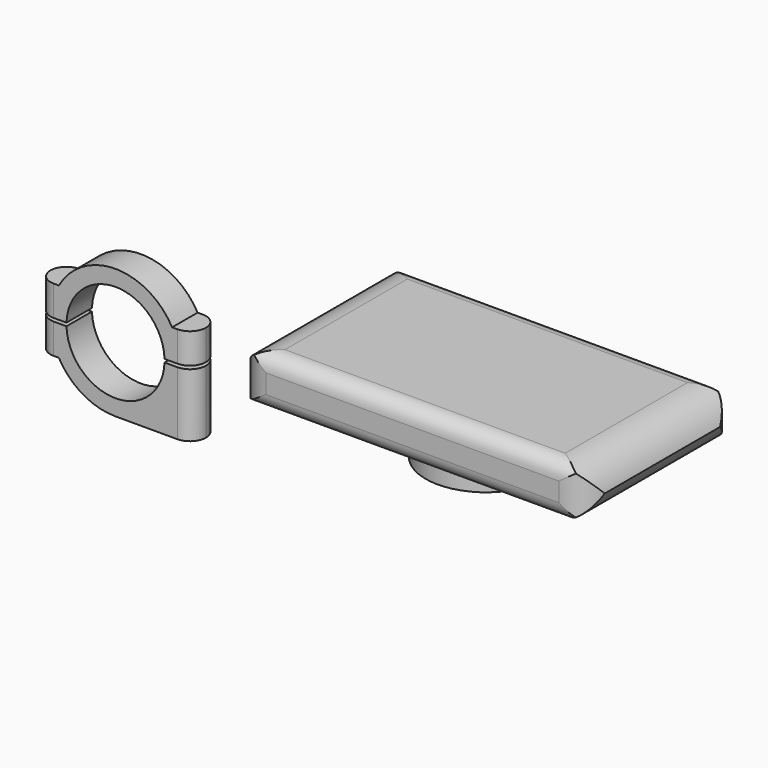
from build123d import *

# Parameters (mm, degrees)
F1_DEPTH       = 5
F2_R           = 1.5
F3_DEPTH       = 25
F4_R           = 2.75
F4_R_2         = 1.5
F5_DEPTH       = 5
F6_R           = 4.99999
F6_2_R         = 4.99999
F7_R           = 1.5
F8_DEPTH       = 16.8
F9_R           = 2.75
F10_DEPTH      = 5
F10_DEPTH_BACK = 10.6
F12_DEPTH      = 8
F13_T1_DEPTH   = 117
F14_T1_DEPTH   = 98
F16_R          = 19
F17_DEPTH      = 6


# Not quite as in the source:
# - a fillet or chamfer that OpenCascade refuses, or shapes differently, is made with other operations: its cross-section is extruded or revolved along the edge and cut away or added
# - a fillet or chamfer is up to 0.001 mm smaller than in the source, because OpenCascade refuses the exact size
# - a feature names something its author has since deleted; it is built from what else it names


with BuildPart() as f1:
    # F0 (on Front) → F1 (new body, symmetric)
    with BuildSketch(Plane.XZ):
        with BuildLine():
            ThreePointArc((20.3938716285, 0.5), (19.6695343093, 5.410122), (17.7808886167, 10))
            ThreePointArc((17.7808886167, 10), (0, 20.4), (-17.7808886167, 10))
            ThreePointArc((-17.7808886167, 10), (-19.6695343093, 5.410122), (-20.3938716285, 0.5))
            Line((-20.3938716285, 0.5), (-15.3918809767, 0.5))
            ThreePointArc((-15.3918809767, 0.5), (0, 15.4), (15.3918809767, 0.5))
            Line((15.3918809767, 0.5), (20.3938716285, 0.5))
        make_face()
        with BuildLine():
            Line((24.4, 10), (17.7808886167, 10))
            ThreePointArc((17.7808886167, 10), (19.6695343093, 5.410122), (20.3938716285, 0.5))
            Line((20.3938716285, 0.5), (24.4, 0.5))
            Line((24.4, 0.5), (24.4, 10))
        make_face()
        with BuildLine():
            ThreePointArc((-20.3938716285, 0.5), (-19.6695343093, 5.410122), (-17.7808886167, 10))
            Line((-17.7808886167, 10), (-24.4, 10))
            Line((-24.4, 10), (-24.4, 0.5))
            Line((-24.4, 0.5), (-20.3938716285, 0.5))
        make_face()
    extrude(amount=F1_DEPTH, both=True)


with BuildPart() as f1b:
    # F0 (on Front) → F1, piece 2 (new body, symmetric)
    with BuildSketch(Plane.XZ):
        with BuildLine():
            Line((-15.3918809767, -0.5), (-20.3938716285, -0.5))
            ThreePointArc((-20.3938716285, -0.5), (-19.6695343093, -5.410122), (-17.7808886167, -10))
            ThreePointArc((-17.7808886167, -10), (-10.2995145517, -17.6090885624), (0, -20.4))
            ThreePointArc((0, -20.4), (14.2471049691, -14.6006849154), (20.3938716285, -0.5))
            Line((20.3938716285, -0.5), (15.3918809767, -0.5))
            ThreePointArc((15.3918809767, -0.5), (0, -15.4), (-15.3918809767, -0.5))
        make_face()
        with BuildLine():
            Line((24.4, -0.5), (20.3938716285, -0.5))
            ThreePointArc((20.3938716285, -0.5), (14.2471049691, -14.6006849154), (0, -20.4))
            Line((0, -20.4), (24.4, -20.4))
            Line((24.4, -20.4), (24.4, -0.5))
        make_face()
        with BuildLine():
            ThreePointArc((-17.7808886167, -10), (-19.6695343093, -5.410122), (-20.3938716285, -0.5))
            Line((-20.3938716285, -0.5), (-24.4, -0.5))
            Line((-24.4, -0.5), (-24.4, -10))
            Line((-24.4, -10), (-17.7808886167, -10))
        make_face()
    extrude(amount=F1_DEPTH, both=True)


with BuildPart() as f3_tool:
    # F2 (on face) → F3 (new body)
    with BuildSketch(Plane(origin=(0, 0, -20.4), x_dir=(1, 0, 0), z_dir=(0, 0, -1))):
        with Locations((19.9, 0)):
            Circle(F2_R)
    extrude(amount=-F3_DEPTH)


with BuildPart() as f1_1:
    add(f1.part)

    # F3: cut by f3_tool
    add(f3_tool.part, mode=Mode.SUBTRACT)

    # F6 (radius 5 in the source; OpenCascade refuses exactly that, so slightly less here)
    f6_edges = [f1_1.edges().sort_by_distance(p)[0] for p in [
        (-24.4, -5, 5.25),
        (-24.4, 5, 5.25),
        (24.4, -5, 5.25),
        (24.4, 5, 5.25),
    ]]
    fillet(f6_edges, radius=F6_R)


with BuildPart() as f1b_1:
    add(f1b.part)

    # F3: cut by f3_tool
    add(f3_tool.part, mode=Mode.SUBTRACT)

    # F4 (on face) → F5 (cut)
    with BuildSketch(Plane(origin=(0, 0, -20.4), x_dir=(1, 0, 0), z_dir=(0, 0, -1))):
        with Locations((19.9, 0)):
            Circle(F4_R)
        with Locations((19.9, 0)):
            Circle(F4_R_2, mode=Mode.SUBTRACT)
    extrude(amount=-F5_DEPTH, mode=Mode.SUBTRACT)

    # F6#2 (radius 5 in the source; OpenCascade refuses exactly that, so slightly less here)
    f6_2_edges = [f1b_1.edges().sort_by_distance(p)[0] for p in [
        (-24.4, -5, -5.25),
        (-24.4, 5, -5.25),
        (24.4, -5, -10.45),
        (24.4, 5, -10.45),
    ]]
    fillet(f6_2_edges, radius=F6_2_R)


with BuildPart() as f8_tool:
    # F7 (on face) → F8 (new body)
    with BuildSketch(Plane(origin=(0, 0, -10), x_dir=(1, 0, 0), z_dir=(0, 0, -1))):
        with Locations((-19.9, 0)):
            Circle(F7_R)
    extrude(amount=-F8_DEPTH)


with BuildPart() as f1_2:
    add(f1_1.part)

    # F8: cut by f8_tool
    add(f8_tool.part, mode=Mode.SUBTRACT)


with BuildPart() as f1b_2:
    add(f1b_1.part)

    # F8: cut by f8_tool
    add(f8_tool.part, mode=Mode.SUBTRACT)

    # F9 (on face) → F10 (cut, two sides)
    with BuildSketch(Plane(origin=(0, 0, -10), x_dir=(1, 0, 0), z_dir=(0, 0, -1))) as f10_sk:
        with Locations((-19.9, 0)):
            Circle(F9_R)
    extrude(amount=-F10_DEPTH, mode=Mode.SUBTRACT)
    extrude(f10_sk.sketch, amount=F10_DEPTH_BACK, mode=Mode.SUBTRACT)


with BuildPart() as f12:
    # F11 (on Top) → F12 (new body, symmetric)
    with BuildSketch(Plane.XY):
        with BuildLine():
            Line((42.4, 1), (134.4, 1))
            ThreePointArc((134.4, 1), (141.4710678119, 3.9289321881), (144.4, 11))
            Line((144.4, 11), (144.4, 49))
            ThreePointArc((144.4, 49), (141.4710678119, 56.0710678119), (134.4, 59))
            Line((134.4, 59), (42.4, 59))
            ThreePointArc((42.4, 59), (35.3289321881, 56.0710678119), (32.4, 49))
            Line((32.4, 49), (32.4, 11))
            ThreePointArc((32.4, 11), (35.3289321881, 3.9289321881), (42.4, 1))
        make_face()
    extrude(amount=F12_DEPTH, both=True)

    # F13: fillet of radius 5 on 4 edges, made by hand

    # F13_s2 → F13_t1 (cut)
    with BuildSketch(Plane.YZ.offset(29.9)):
        with BuildLine():
            ThreePointArc((1, 3), (2.4644660941, 6.5355339059), (6, 8))
            Line((6, 8), (1, 8))
            Line((1, 8), (1, 3))
        make_face()
        with BuildLine():
            ThreePointArc((59, 3), (57.5355339059, 6.5355339059), (54, 8))
            Line((54, 8), (59, 8))
            Line((59, 8), (59, 3))
        make_face()
        with BuildLine():
            ThreePointArc((1, -3), (2.4644660941, -6.5355339059), (6, -8))
            Line((6, -8), (1, -8))
            Line((1, -8), (1, -3))
        make_face()
        with BuildLine():
            ThreePointArc((59, -3), (57.5355339059, -6.5355339059), (54, -8))
            Line((54, -8), (59, -8))
            Line((59, -8), (59, -3))
        make_face()
    extrude(amount=F13_T1_DEPTH, mode=Mode.SUBTRACT)

    # F14: fillet of radius 12 on 3 edges, made by hand

    # F14_s2 → F14_t1 (cut)
    with BuildSketch(Plane.XZ.offset(-79)):
        with BuildLine():
            ThreePointArc((132.4, 8), (140.8852813742, 4.4852813742), (144.4, -4))
            Line((144.4, -4), (144.4, 8))
            Line((144.4, 8), (132.4, 8))
        make_face()
        with BuildLine():
            ThreePointArc((32.4, -4), (35.9147186258, 4.4852813742), (44.4, 8))
            Line((44.4, 8), (32.4, 8))
            Line((32.4, 8), (32.4, -4))
        make_face()
        with BuildLine():
            ThreePointArc((132.4, -8), (140.8852813742, -4.4852813742), (144.4, 4))
            Line((144.4, 4), (144.4, -8))
            Line((144.4, -8), (132.4, -8))
        make_face()
    extrude(amount=F14_T1_DEPTH, mode=Mode.SUBTRACT)


with BuildPart() as f17:
    # F16 (on offset) → F17 (new body)
    with BuildSketch(Plane(origin=(0, 0, -11), x_dir=(1, 0, 0), z_dir=(0, 0, -1))):
        with Locations((88.4, -30)):
            Circle(F16_R)
    extrude(amount=F17_DEPTH)


solid = Compound([f1_2.part, f1b_2.part, f12.part, f17.part])
